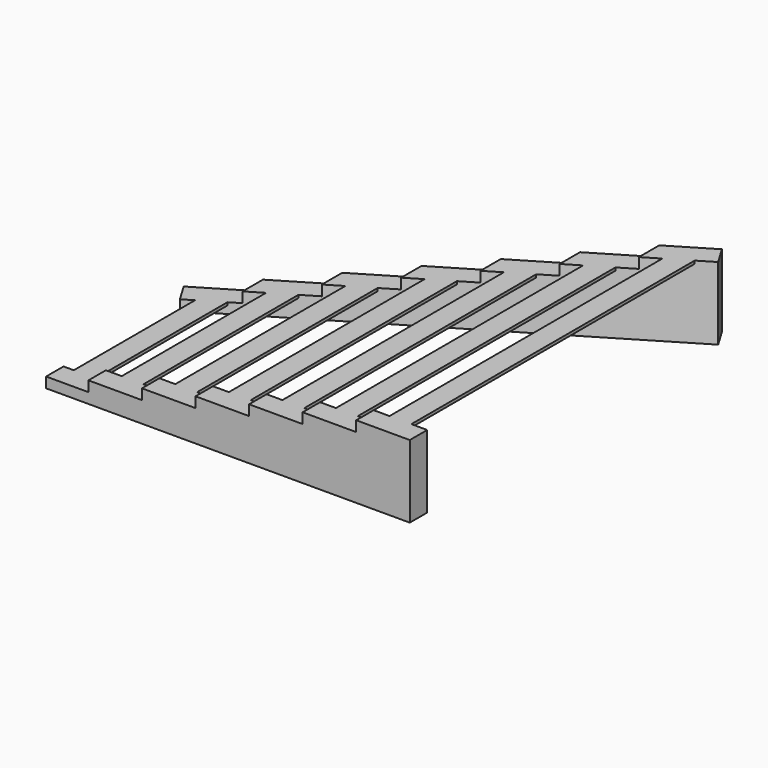
from build123d import *

# Parameters (mm, degrees)
F0_W     = 50
F0_H     = 3
F1_DEPTH = 10
F3_DEPTH = 55.5734787771
F4_W     = 3
F4_H     = 0.4
F5_REACH = 58.6000279672


with BuildPart() as f1:
    # F0 (on Top) → F1 (new body)
    with BuildSketch(Plane.XY):
        Rectangle(F0_W, F0_H)
    extrude(amount=F1_DEPTH)


with BuildPart() as f1b:
    # F0 (on Top) → F1, piece 2 (new body)
    with BuildSketch(Plane.XY):
        Polygon((-26.5434872663, 24.0724787771), (-25, 21.5), (25, 51.5), (23.4565127337, 54.0724787771), align=None)
    extrude(amount=F1_DEPTH)


with BuildPart() as f3_tool:
    # F2 (on face) → F3 (new body, through all)
    with BuildSketch(Plane.XZ.offset(1.5)):
        Polygon((17.6366446762, 10), (-26.5434872663, 10), (-26.5434872663, 1.4285714286), (-19.1801319425, 1.4285714286), (-19.1801319425, 2.8571428571), (-11.8167766188, 2.8571428571), (-11.8167766188, 4.2857142857), (-4.453421295, 4.2857142857), (-4.453421295, 5.7142857143), (2.9099340287, 5.7142857143), (2.9099340287, 7.1428571429), (10.2732893525, 7.1428571429), (10.2732893525, 8.5714285714), (17.6366446762, 8.5714285714), align=None)
    extrude(amount=-F3_DEPTH)


with BuildPart() as f1_1:
    add(f1.part)

    # F3: cut by f3_tool
    add(f3_tool.part, mode=Mode.SUBTRACT)



with BuildPart() as f1b_1:
    add(f1b.part)

    # F3: cut by f3_tool
    add(f3_tool.part, mode=Mode.SUBTRACT)


with BuildPart() as f1_2:
    add(f1_1.part)

    add(f1b_1.part)  # F5 merges F1b
    f5_end = f1_2.faces().sort_by_distance((5.616262324, 43.3683285313, 3.4924250952))[0]
    # F4 (on face) → F5 (join, up to a face of the model that its end follows)
    with BuildSketch(Plane.XZ.offset(1.5)):
        with Locations((-22.0900659713, 1.2285714286)):
            Rectangle(F4_W, F4_H)
        with Locations((-15.4984542807, 2.6571428571)):
            Rectangle(F4_W, F4_H)
        with Locations((-8.1350989569, 4.0857142857)):
            Rectangle(F4_W, F4_H)
        with Locations((-0.7717436331, 5.5142857143)):
            Rectangle(F4_W, F4_H)
        with Locations((6.5916116906, 6.9428571429)):
            Rectangle(F4_W, F4_H)
        with Locations((13.9549670144, 8.3714285714)):
            Rectangle(F4_W, F4_H)
        with Locations((21.3183223381, 9.8)):
            Rectangle(F4_W, F4_H)
    f5_long = extrude(amount=-F5_REACH, mode=Mode.PRIVATE)
    add(split(f5_long, bisect_by=f5_end, keep=Keep.BOTTOM, mode=Mode.PRIVATE))


solid = f1_2.part
